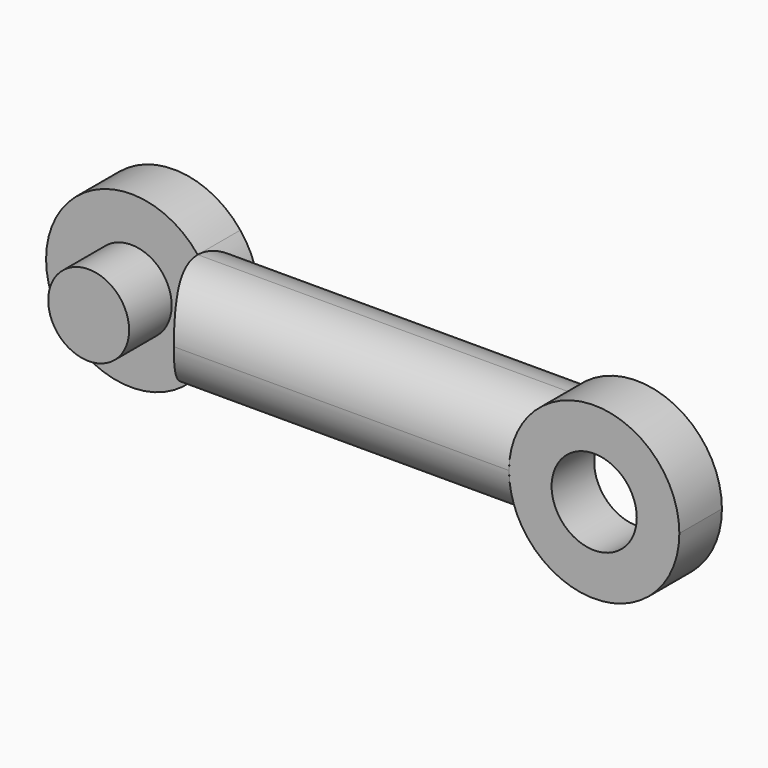
from build123d import *

# Parameters (mm, degrees)
F1_DEPTH = 6.35
F2_R     = 6.3499
F0_R     = 5.08
F3_DEPTH = 6.35
F0_R_2   = 4.826
F4_DEPTH = 6.35
F5_DEPTH = 6.35


# Not quite as in the source:
# - a fillet or chamfer is up to 0.001 mm smaller than in the source, because OpenCascade refuses the exact size


with BuildPart() as f1:
    # F0 (on Front) → F1 (new body, symmetric)
    with BuildSketch(Plane.XZ):
        with BuildLine():
            Line((22.225, 6.35), (-22.225, 6.35))
            ThreePointArc((-22.225, 6.35), (-20.5695407024, 3.3649028089), (-19.996147458, 0))
            ThreePointArc((-19.996147458, 0), (-20.5695407024, -3.3649028089), (-22.225, -6.35))
            Line((-22.225, -6.35), (22.225, -6.35))
            ThreePointArc((22.225, -6.35), (19.996147458, 0), (22.225, 6.35))
        make_face()
    extrude(amount=F1_DEPTH, both=True)

    # F2 (radius 6.35 in the source; OpenCascade refuses exactly that, so slightly less here)
    f2_edges = [f1.edges().sort_by_distance(p)[0] for p in [
        (0, -6.35, 6.35),
        (0, 6.35, 6.35),
        (0, -6.35, -6.35),
        (0, 6.35, -6.35),
    ]]
    fillet(f2_edges, radius=F2_R)

    # F0 (on Front) → F3 (join)
    with BuildSketch(Plane.XZ):
        with BuildLine():
            ThreePointArc((40.316147458, 0), (33.5210502669, 9.5866067556), (22.225, 6.35))
            Line((22.225, 6.35), (22.225, -6.35))
            ThreePointArc((22.225, -6.35), (33.5210502669, -9.5866067556), (40.316147458, 0))
        make_face()
        with Locations((30.156147458, 0)):
            Circle(F0_R, mode=Mode.SUBTRACT)
        with BuildLine():
            Line((22.225, -6.35), (22.225, 6.35))
            ThreePointArc((22.225, 6.35), (19.996147458, 0), (22.225, -6.35))
        make_face()
    extrude(amount=F3_DEPTH)

    # F0 (on Front) → F4 (join)
    with BuildSketch(Plane.XZ):
        with BuildLine():
            Line((-22.225, -6.35), (-22.225, 6.35))
            ThreePointArc((-22.225, 6.35), (-40.316147458, 0), (-22.225, -6.35))
        make_face()
        with Locations((-30.156147458, 0)):
            Circle(F0_R_2, mode=Mode.SUBTRACT)
        with BuildLine():
            ThreePointArc((-19.996147458, 0), (-20.5695407024, 3.3649028089), (-22.225, 6.35))
            Line((-22.225, 6.35), (-22.225, -6.35))
            ThreePointArc((-22.225, -6.35), (-20.5695407024, -3.3649028089), (-19.996147458, 0))
        make_face()
    extrude(amount=-F4_DEPTH)

    # F0 (on Front) → F5 (join, symmetric)
    with BuildSketch(Plane.XZ):
        with Locations((-30.156147458, 0)):
            Circle(F0_R_2)
    extrude(amount=F5_DEPTH, both=True)


solid = f1.part
